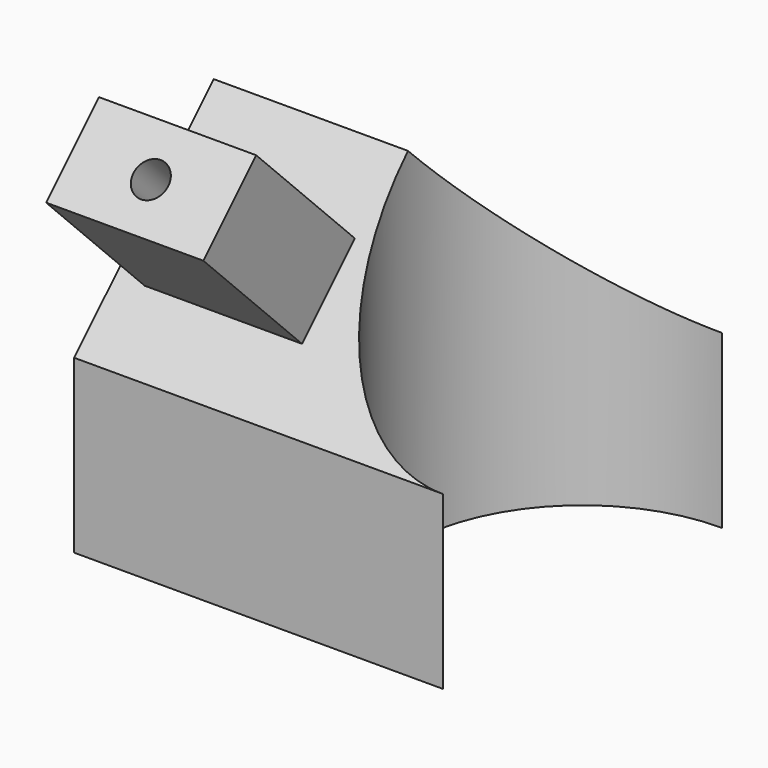
from build123d import *

# Parameters (mm, degrees)
F1_DEPTH    = 10
F2_T1_DEPTH = 36.6968120455
F3_W        = 4.5079379342
F3_H        = 2.6771172415
F4_DEPTH    = 5
F6_D        = 1
F6_DEPTH    = 10
F6_TIP      = 0.3004303095


# Not quite as in the source:
# - a fillet or chamfer that OpenCascade refuses, or shapes differently, is made with other operations: its cross-section is extruded or revolved along the edge and cut away or added


with BuildPart() as f1:
    # F0 (on Top) → F1 (new body)
    with BuildSketch(Plane.XY):
        with BuildLine():
            ThreePointArc((0, -5), (-5, 0), (0, 5))
            Line((0, 5), (-10.5685128878, 5))
            Line((-10.5685128878, 5), (-10.5685128878, -5))
            Line((-10.5685128878, -5), (0, -5))
        make_face()
    extrude(amount=F1_DEPTH)

    # F2: chamfer of 5.08 on 2 edges, made by hand

    # F2_s2 → F2_t1 (cut)
    with BuildSketch(Plane.YZ.offset(-23.6326624666)):
        Polygon((-5, 4.92), (0.08, 10), (-5, 10), align=None)
        Polygon((5, 4.92), (-0.08, 10), (5, 10), align=None)
    extrude(amount=F2_T1_DEPTH, mode=Mode.SUBTRACT)

    # F3 (on face) → F4 (join)
    with BuildSketch(Plane(origin=(0, -4.96, 4.96), x_dir=(1, 0, 0), z_dir=(0, -0.7071067812, 0.7071067812))):
        with Locations((-7.4802257586, 3.3821087563)):
            Rectangle(F3_W, F3_H)
    extrude(amount=F4_DEPTH)

    # F6
    with Locations(Plane(origin=(0, -8.4955339059, 8.4955339059), x_dir=(1, 0, 0), z_dir=(0, -0.7071067812, 0.7071067812))):
        with Locations((-7.4782376178, 3.3632300328)):
            Hole(F6_D / 2, depth=F6_DEPTH)
            with Locations((0, 0, -(F6_DEPTH + F6_TIP / 2))):  # 118° drill point
                Cone(0, F6_D / 2, F6_TIP, mode=Mode.SUBTRACT)


solid = f1.part
